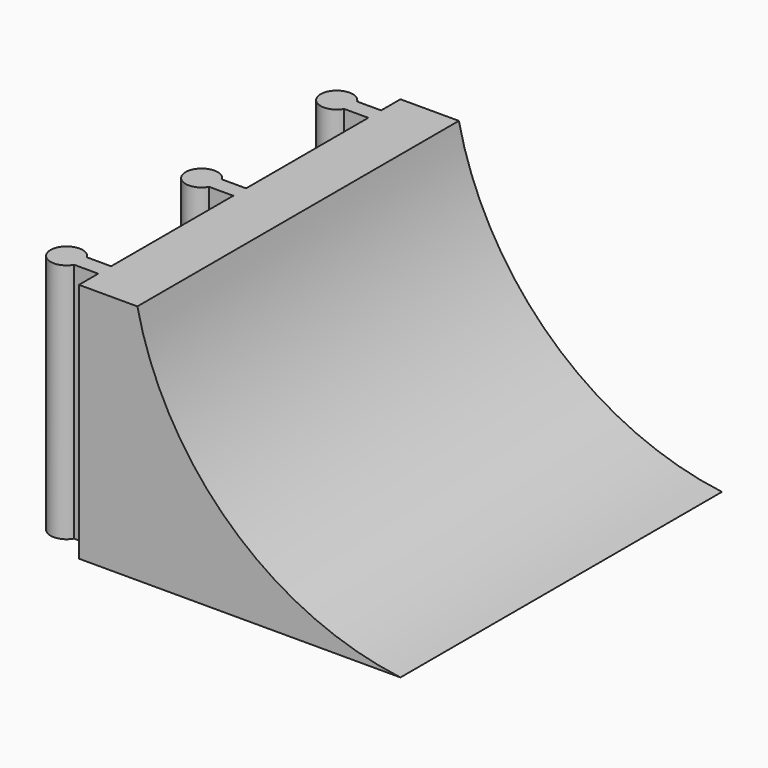
from build123d import *

# Parameters (mm, degrees)
F0_W     = 101.6
F0_H     = 101.6
F1_DEPTH = 76.2
F3_DEPTH = 101.6
F4_W     = 63.5649934411
F4_H     = 88.8701714575
F5_DEPTH = 7.62
F7_DEPTH = 25.4
F8_W     = 7.62
F8_H     = 5.08
F9_DEPTH = 76.2


# Not quite as in the source:
# - a feature names something its author has since deleted; it is built from what else it names


with BuildPart() as f1:
    # F0 (on Top) → F1 (new body)
    with BuildSketch(Plane.XY):
        with Locations((-18.5535050273, 1.2484980512)):
            Rectangle(F0_W, F0_H)
    extrude(amount=F1_DEPTH)

    # F2 (on face) → F3 (cut)
    with BuildSketch(Plane.XZ.offset(49.5515019488)):
        with BuildLine():
            Line((32.2464949727, 76.2), (-50.8901812136, 76.2))
            ThreePointArc((-50.8901812136, 76.2), (-21.4414456403, 24.8771198137), (32.2464949727, 0))
            Line((32.2464949727, 0), (32.2464949727, 76.2))
        make_face()
    extrude(amount=-F3_DEPTH, mode=Mode.SUBTRACT)

    # F4 (on face) → F5 (join)
    with BuildSketch(Plane(origin=(0, 0, 0), x_dir=(1, 0, 0), z_dir=(0, 0, -1))):
        with Locations((-31.7824967206, -2.1479185671)):
            Rectangle(F4_W, F4_H)
    extrude(amount=-F5_DEPTH)

    # F6 (on face) → F7 (join)
    with BuildSketch(Plane.XZ.offset(49.5515019488)):
        with BuildLine():
            Line((-69.3535050273, 76.2), (-69.3535050273, 0))
            Line((-69.3535050273, 0), (32.2464949727, 0))
            ThreePointArc((32.2464949727, 0), (-21.4414456403, 24.8771198137), (-50.8901812136, 76.2))
            Line((-50.8901812136, 76.2), (-69.3535050273, 76.2))
        make_face()
    extrude(amount=F7_DEPTH)

    # F8 (on face) → F9 (join)
    with BuildSketch(Plane(origin=(0, 0, 0), x_dir=(1, 0, 0), z_dir=(0, 0, -1))):
        with BuildLine():
            Line((-76.9735050273, -44.4284980512), (-76.9735050273, -39.3484980512))
            ThreePointArc((-76.9735050273, -39.3484980512), (-86.4529140785, -41.8884980512), (-76.9735050273, -44.4284980512))
        make_face()
        with Locations((-73.1635050273, -41.8884980512)):
            Rectangle(F8_W, F8_H)
        with BuildLine():
            Line((-76.9735050273, 8.9115019488), (-76.9735050273, 13.9915019488))
            ThreePointArc((-76.9735050273, 13.9915019488), (-86.4529140785, 11.4515019488), (-76.9735050273, 8.9115019488))
        make_face()
        with Locations((-73.1635050273, 11.4515019488)):
            Rectangle(F8_W, F8_H)
        with Locations((-73.1635050273, 64.7915019488)):
            Rectangle(F8_W, F8_H)
        with BuildLine():
            ThreePointArc((-76.9735050273, 67.3315019488), (-86.4529140785, 64.7915019488), (-76.9735050273, 62.2515019488))
            Line((-76.9735050273, 62.2515019488), (-76.9735050273, 67.3315019488))
        make_face()
    extrude(amount=-F9_DEPTH)


solid = f1.part
